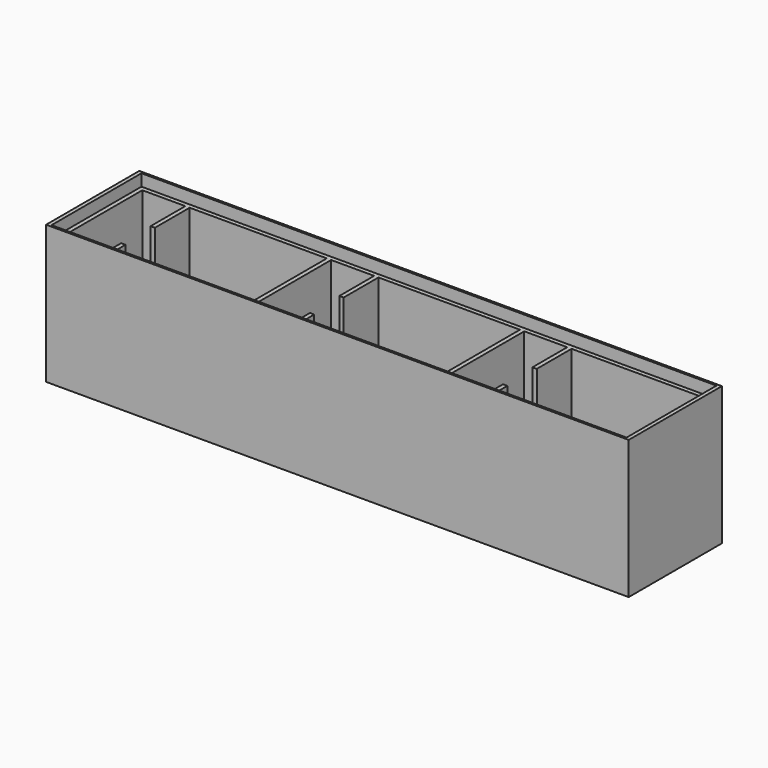
from build123d import *

# Parameters (mm, degrees)
F0_W     = 12192
F0_H     = 2438
F0_W_2   = 12032
F0_H_2   = 2352
F1_DEPTH = 2896
F2_DEPTH = 99
F3_W     = 90
F3_H     = 90
F3_W_2   = 2871
F3_H_2   = 910
F3_H_3   = 2172
F3_H_4   = 492
F3_W_3   = 900
F3_W_4   = 2961
F4_DEPTH = 2550


with BuildPart() as f1:
    # F0 (on Top) → F1 (new body)
    with BuildSketch(Plane.XY):
        Rectangle(F0_W, F0_H)
        Rectangle(F0_W_2, F0_H_2, mode=Mode.SUBTRACT)
    extrude(amount=F1_DEPTH)

    # F0 (on Top) → F2 (join)
    with BuildSketch(Plane.XY):
        Rectangle(F0_W_2, F0_H_2)
    extrude(amount=F2_DEPTH)

    # F3 (on face) → F4 (join)
    with BuildSketch(Plane.XY.offset(99)):
        Polygon((-5026, 1086), (-5026, 1176), (-6016, 1176), (-6016, 1086), (-5926, 1086), align=None)
        with Locations((-4981, 1131)):
            Rectangle(F3_W, F3_H)
        with Locations((-3500.5, 1131)):
            Rectangle(F3_W_2, F3_H)
        with Locations((-4981, 631)):
            Rectangle(F3_W, F3_H_2)
        with Locations((-5971, 0)):
            Rectangle(F3_W, F3_H_3)
        Polygon((-5026, -1176), (-5026, -1086), (-5926, -1086), (-6016, -1086), (-6016, -1176), align=None)
        with Locations((-4981, -840)):
            Rectangle(F3_W, F3_H_4)
        with Locations((-4981, -1131)):
            Rectangle(F3_W, F3_H)
        with Locations((-3500.5, -1131)):
            Rectangle(F3_W_2, F3_H)
        with Locations((-2020, 0)):
            Rectangle(F3_W, F3_H_3)
        with Locations((-2020, 1131)):
            Rectangle(F3_W, F3_H)
        with Locations((-1525, 1131)):
            Rectangle(F3_W_3, F3_H)
        with Locations((-1030, 1131)):
            Rectangle(F3_W, F3_H)
        with Locations((495.5, 1131)):
            Rectangle(F3_W_4, F3_H)
        with Locations((-1030, 631)):
            Rectangle(F3_W, F3_H_2)
        with Locations((-1525, -1131)):
            Rectangle(F3_W_3, F3_H)
        with Locations((-2020, -1131)):
            Rectangle(F3_W, F3_H)
        with Locations((-1030, -840)):
            Rectangle(F3_W, F3_H_4)
        with Locations((-1030, -1131)):
            Rectangle(F3_W, F3_H)
        with Locations((495.5, -1131)):
            Rectangle(F3_W_4, F3_H)
        with Locations((2021, 0)):
            Rectangle(F3_W, F3_H_3)
        with Locations((2021, 1131)):
            Rectangle(F3_W, F3_H)
        with Locations((2021, -1131)):
            Rectangle(F3_W, F3_H)
        with Locations((2516, -1131)):
            Rectangle(F3_W_3, F3_H)
        with Locations((3011, -1131)):
            Rectangle(F3_W, F3_H)
        Polygon((5926, -1086), (3056, -1086), (3056, -1176), (6016, -1176), (6016, -1086), align=None)
        with Locations((3011, -840)):
            Rectangle(F3_W, F3_H_4)
        with Locations((3011, 631)):
            Rectangle(F3_W, F3_H_2)
        with Locations((3011, 1131)):
            Rectangle(F3_W, F3_H)
        with Locations((2516, 1131)):
            Rectangle(F3_W_3, F3_H)
        Polygon((6016, 1176), (3056, 1176), (3056, 1086), (5926, 1086), (6016, 1086), align=None)
        with Locations((5971, 0)):
            Rectangle(F3_W, F3_H_3)
    extrude(amount=F4_DEPTH)


solid = f1.part
